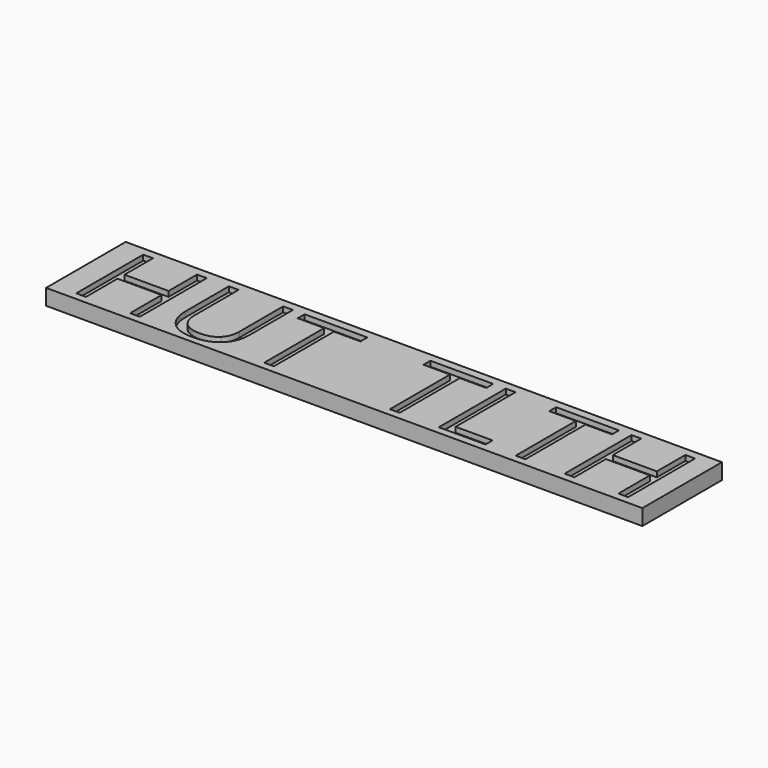
from build123d import *

# Parameters (mm, degrees)
F0_W         = 113
F0_H         = 18.85
F1_DEPTH     = 3
F0_TEXT_SIZE = 22.2222222222
F2_DEPTH     = 2


# Not quite as in the source:
# - Text() gives the source's letters only with a copy of the font that has no kerning and outlines rounded to 1/6400 em; it was checked with that copy


with BuildPart() as f1:
    # F0 (on Top) → F1 (new body)
    with BuildSketch(Plane.XY):
        with Locations((-23.0842265031, 25.8628010448)):
            Rectangle(F0_W, F0_H)
        Polygon((-62.9625320587, 33.7273843782), (-62.9625320587, 17.8628010448), (-64.8062820587, 17.8628010448), (-64.8062820587, 25.3280788226), (-73.1639209476, 25.3280788226), (-73.1639209476, 17.8628010448), (-75.0076709476, 17.8628010448), (-75.0076709476, 33.7273843782), (-73.1639209476, 33.7273843782), (-73.1639209476, 26.9773843782), (-64.8062820587, 26.9773843782), (-64.8062820587, 33.7273843782), align=None, mode=Mode.SUBTRACT)
        with BuildLine():
            Line((-48.4764209476, 33.7273843782), (-46.6326709476, 33.7273843782))
            Line((-46.6326709476, 33.7273843782), (-46.6326709476, 23.4634954893))
            add(Edge.make_bspline(
                [(-46.6326709476, 23.4634954893), (-46.6326709476, 20.7482177115), (-48.2715598365, 19.1961343782)],
                knots=[0, 0, 0, 1, 1, 1], degree=2))
            add(Edge.make_bspline(
                [(-48.2715598365, 19.1961343782), (-49.9104487253, 17.6440510448), (-52.7750320587, 17.6440510448)],
                knots=[0, 0, 0, 1, 1, 1], degree=2))
            add(Edge.make_bspline(
                [(-52.7750320587, 17.6440510448), (-55.639615392, 17.6440510448), (-57.2073237253, 19.208287156)],
                knots=[0, 0, 0, 1, 1, 1], degree=2))
            add(Edge.make_bspline(
                [(-57.2073237253, 19.208287156), (-58.7750320587, 20.7725232671), (-58.7750320587, 23.505162156)],
                knots=[0, 0, 0, 1, 1, 1], degree=2))
            Line((-58.7750320587, 23.505162156), (-58.7750320587, 33.7273843782))
            Line((-58.7750320587, 33.7273843782), (-56.9278098365, 33.7273843782))
            Line((-56.9278098365, 33.7273843782), (-56.9278098365, 23.3766899337))
            add(Edge.make_bspline(
                [(-56.9278098365, 23.3766899337), (-56.9278098365, 21.3905788226), (-55.842740392, 20.3263427115)],
                knots=[0, 0, 0, 1, 1, 1], degree=2))
            add(Edge.make_bspline(
                [(-55.842740392, 20.3263427115), (-54.7576709476, 19.2621066004), (-52.6535042809, 19.2621066004)],
                knots=[0, 0, 0, 1, 1, 1], degree=2))
            add(Edge.make_bspline(
                [(-52.6535042809, 19.2621066004), (-50.6465598365, 19.2621066004), (-49.561490392, 20.3315510448)],
                knots=[0, 0, 0, 1, 1, 1], degree=2))
            add(Edge.make_bspline(
                [(-49.561490392, 20.3315510448), (-48.4764209476, 21.4009954893), (-48.4764209476, 23.3975232671)],
                knots=[0, 0, 0, 1, 1, 1], degree=2))
            Line((-48.4764209476, 23.3975232671), (-48.4764209476, 33.7273843782))
        make_face(mode=Mode.SUBTRACT)
        Polygon((-37.5528098365, 32.0884954893), (-37.5528098365, 17.8628010448), (-39.3965598365, 17.8628010448), (-39.3965598365, 32.0884954893), (-44.420865392, 32.0884954893), (-44.420865392, 33.7273843782), (-32.5285042809, 33.7273843782), (-32.5285042809, 32.0884954893), align=None, mode=Mode.SUBTRACT)
        Polygon((-13.7090598365, 32.0884954893), (-13.7090598365, 17.8628010448), (-15.5528098365, 17.8628010448), (-15.5528098365, 32.0884954893), (-20.577115392, 32.0884954893), (-20.577115392, 33.7273843782), (-8.6847542809, 33.7273843782), (-8.6847542809, 32.0884954893), align=None, mode=Mode.SUBTRACT)
        Polygon((2.547884608, 17.8628010448), (-6.295865392, 17.8628010448), (-6.295865392, 33.7273843782), (-4.452115392, 33.7273843782), (-4.452115392, 19.5329399337), (2.547884608, 19.5329399337), align=None, mode=Mode.SUBTRACT)
        Polygon((10.1208012747, 32.0884954893), (10.1208012747, 17.8628010448), (8.2770512747, 17.8628010448), (8.2770512747, 32.0884954893), (3.2527457191, 32.0884954893), (3.2527457191, 33.7273843782), (15.1451068302, 33.7273843782), (15.1451068302, 32.0884954893), align=None, mode=Mode.SUBTRACT)
        Polygon((29.579134608, 33.7273843782), (29.579134608, 17.8628010448), (27.735384608, 17.8628010448), (27.735384608, 25.3280788226), (19.3777457191, 25.3280788226), (19.3777457191, 17.8628010448), (17.5339957191, 17.8628010448), (17.5339957191, 33.7273843782), (19.3777457191, 33.7273843782), (19.3777457191, 26.9773843782), (27.735384608, 26.9773843782), (27.735384608, 33.7273843782), align=None, mode=Mode.SUBTRACT)
    extrude(amount=F1_DEPTH)

    # F0 (on Top) → F2 (join)
    with BuildSketch(Plane.XY):
        with Locations((-77.1882265031, 17.8628010448)):
            Text('HUT  TLTH', F0_TEXT_SIZE, font='Open Sans', text_align=(TextAlign.LEFT, TextAlign.BOTTOM))
    extrude(amount=F2_DEPTH)


solid = f1.part
